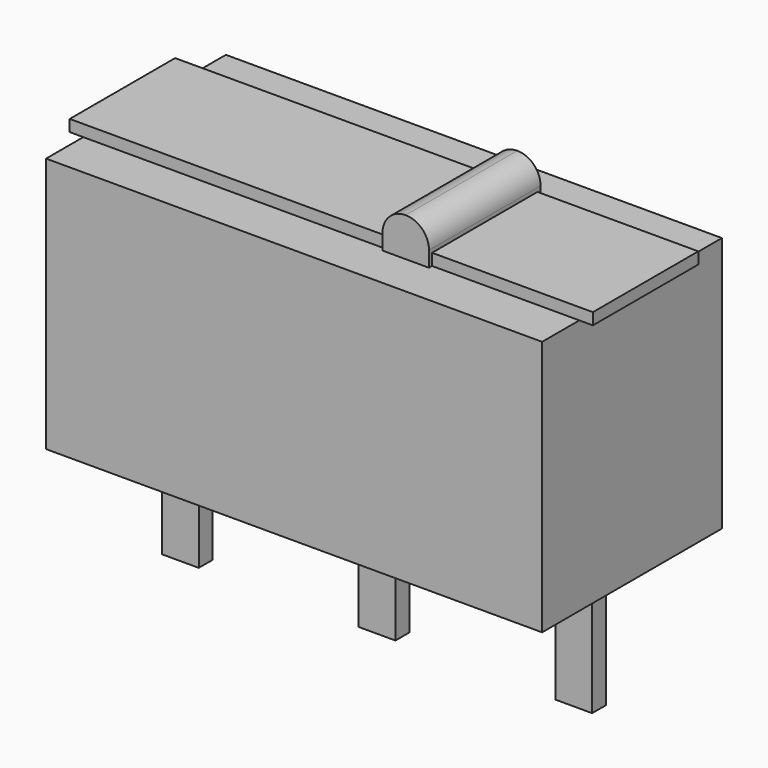
from build123d import *

# Parameters (mm, degrees)
F0_W     = 12.8
F0_H     = 5.8
F1_DEPTH = 6.6
F2_W     = 0.95
F2_H     = 0.45
F3_DEPTH = 3.2
F4_W     = 1.2
F4_H     = 3.6
F5_DEPTH = 1
F6_R     = 0.59999
F7_W     = 13.5
F7_H     = 3.4
F8_DEPTH = 0.3


# Not quite as in the source:
# - a fillet or chamfer is up to 0.001 mm smaller than in the source, because OpenCascade refuses the exact size


with BuildPart() as f1:
    # F0 (on Top) → F1 (new body)
    with BuildSketch(Plane.XY):
        Rectangle(F0_W, F0_H)
    extrude(amount=F1_DEPTH)

    # F2 (on face) → F3 (join)
    with BuildSketch(Plane(origin=(0, 0, 0), x_dir=(1, 0, 0), z_dir=(0, 0, -1))):
        with Locations((-5.075, 0)):
            Rectangle(F2_W, F2_H)
        Rectangle(F2_W, F2_H)
        with Locations((5.075, 0)):
            Rectangle(F2_W, F2_H)
    extrude(amount=F3_DEPTH)

    # F4 (on face) → F5 (join)
    with BuildSketch(Plane.XY.offset(6.6)):
        with Locations((2, 0)):
            Rectangle(F4_W, F4_H)
    extrude(amount=F5_DEPTH)

    # F6 (radius 0.6 in the source; OpenCascade refuses exactly that, so slightly less here)
    f6_edges = [f1.edges().sort_by_distance(p)[0] for p in [
        (1.4, 0, 7.6),
        (2.6, 0, 7.6),
    ]]
    fillet(f6_edges, radius=F6_R)


with BuildPart() as f8:
    # F7 (on face) → F8 (new body)
    with BuildSketch(Plane.XY.offset(6.6)):
        Rectangle(F7_W, F7_H)
    extrude(amount=F8_DEPTH)


solid = Compound([f1.part, f8.part])
